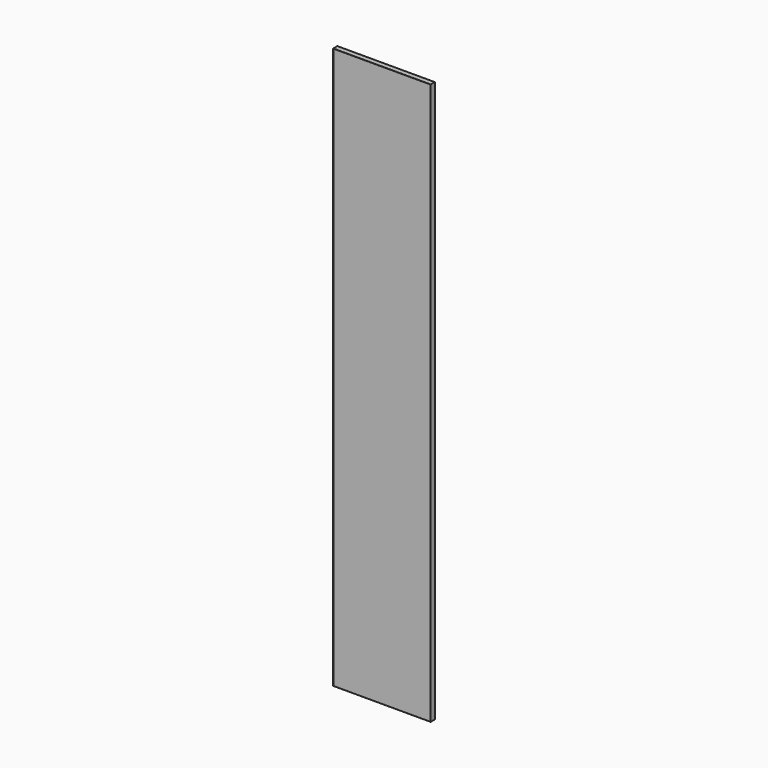
from build123d import *

# Parameters (mm, degrees)
F0_W     = 300
F0_H     = 1728
F1_DEPTH = 16
F2_R     = 0.5
F3_ANGLE = 180


# Not quite as in the source:
# - a feature of the source that left no trace in its solid (it failed there, or was rolled back) is left out


with BuildPart() as f1:
    # F0 (on Front) → F1 (new body)
    with BuildSketch(Plane.XZ):
        with Locations((4.4365953654, 0)):
            Rectangle(F0_W, F0_H)
    extrude(amount=F1_DEPTH)

    # F2
    f2_edges = [f1.edges().sort_by_distance(p)[0] for p in [
        (154.436595, -16, 0),
        (4.436595, -16, 864),
        (-145.563405, -16, 0),
        (4.436595, -16, -864),
    ]]
    fillet(f2_edges, radius=F2_R)


with BuildPart() as f3_1:
    # F3: copy of F1
    add(f1.part.rotate(Axis((154.4365953654, 0, 0), (0, 0, -1)), F3_ANGLE))


solid = f1.part
